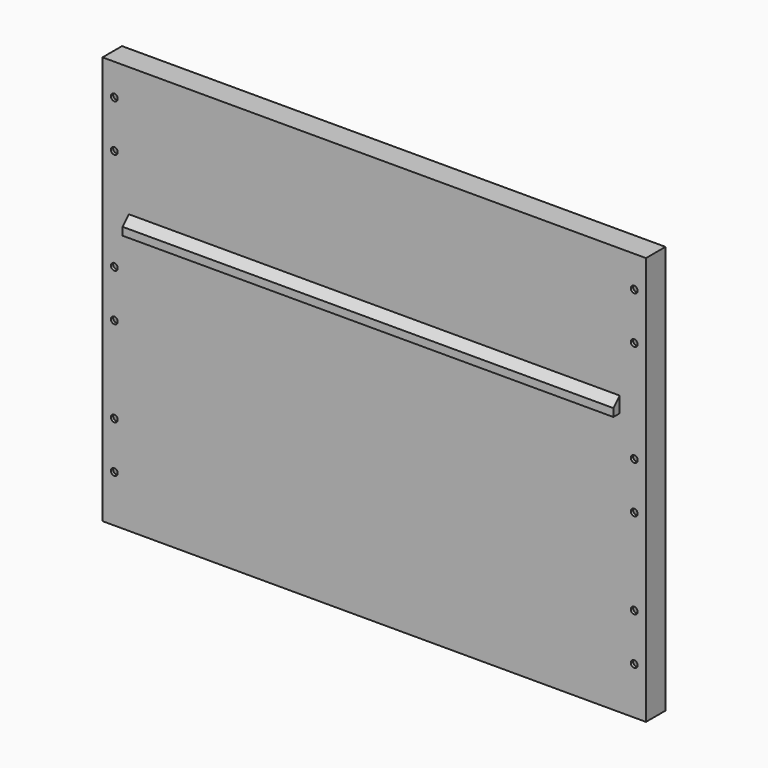
from build123d import *

# Parameters (mm, degrees)
F1_W           = 76.2
F1_H           = 76.2
F1_W_2         = 63.5
F1_H_2         = 63.5
F3_W           = 76.2
F3_H           = 76.2
F3_W_2         = 63.5
F3_H_2         = 63.5
F4_DEPTH       = 802.767
F4_DEPTH_BACK  = 802.767
F5_W           = 1757.934
F5_H           = 2.667
F6_DEPTH       = 660.4
F6_DEPTH_BACK  = 660.4
F7_W           = 19.05
F7_H           = 19.05
F8_DEPTH       = 793.75
F9_W           = 6.35
F9_H           = 25.4
F10_REACH      = 496.0827207226
F11_R          = 11.1125
F12_DEPTH      = 104.268
F13_R          = 9.525
F14_DEPTH      = 76.2
F15_R          = 6.35
F16_DEPTH      = 177.8
F16_DEPTH_BACK = 177.8


# Not quite as in the source:
# - an extrude ends at something that could not be found from the text; its depth is read off the source's solid


with BuildPart() as f2:
    # F2: sweep along a path in F0
    with BuildLine(Plane.XZ) as f2_path:
        Line((-878.967, 660.4), (878.967, 660.4))
        Line((878.967, 660.4), (878.967, -660.4))
        Line((878.967, -660.4), (-878.967, -660.4))
        Line((-878.967, -660.4), (-878.967, 660.4))
    # F1 (on Top) → F2 (sweep)
    with BuildSketch(Plane.XY):
        with Locations((-840.867, -38.1)):
            Rectangle(F1_W, F1_H)
        with Locations((-840.867, -38.1)):
            Rectangle(F1_W_2, F1_H_2, mode=Mode.SUBTRACT)
    sweep(path=f2_path.line, transition=Transition.RIGHT)

    # F3 (on Right) → F4 (join, two sides)
    with BuildSketch(Plane.YZ) as f4_sk:
        with Locations((-38.1, 215.9)):
            Rectangle(F3_W, F3_H)
        with Locations((-38.1, 215.9)):
            Rectangle(F3_W_2, F3_H_2, mode=Mode.SUBTRACT)
        with Locations((-38.1, -215.9)):
            Rectangle(F3_W, F3_H)
        with Locations((-38.1, -215.9)):
            Rectangle(F3_W_2, F3_H_2, mode=Mode.SUBTRACT)
    extrude(amount=-F4_DEPTH)
    extrude(f4_sk.sketch, amount=F4_DEPTH_BACK)

    # F5 (on Top) → F6 (join, two sides)
    with BuildSketch(Plane.XY) as f6_sk:
        with Locations((0, -77.5335)):
            Rectangle(F5_W, F5_H)
    extrude(amount=F6_DEPTH)
    extrude(f6_sk.sketch, amount=-F6_DEPTH_BACK)

    # F7 (on Right) → F8 (join, symmetric)
    with BuildSketch(Plane.YZ):
        Polygon((-78.867, 190.5), (-78.867, 215.9), (-102.5499750297, 215.9), (-104.267, 215.9), (-104.267, 190.5), align=None)
        with Locations((-91.567, 203.2)):
            Rectangle(F7_W, F7_H, mode=Mode.SUBTRACT)
        Polygon((-104.267, 215.9), (-102.5499750297, 215.9), (-78.867, 239.5829750297), (-78.867, 241.3), align=None)
    extrude(amount=F8_DEPTH, both=True)

    f10_end = Plane(origin=(0, -90.7084875148, 227.7414875149), x_dir=(0, 0.7071067812, 0.7071067812), z_dir=(0, 0.7071067812, -0.7071067812))
    # F9 (on face) → F10 (join, up to a plane its end follows)
    with BuildSketch(Plane(origin=(0, 0, 190.5000000001), x_dir=(1, 0, 0), z_dir=(0, 0, -1))):
        with Locations((790.575, 91.567)):
            Rectangle(F9_W, F9_H)
        with Locations((-790.575, 91.567)):
            Rectangle(F9_W, F9_H)
    f10_long = extrude(amount=-F10_REACH, mode=Mode.PRIVATE)
    add(split(f10_long, bisect_by=f10_end, keep=Keep.TOP, mode=Mode.PRIVATE))

    # F11 (on Front) → F12 (cut, through all)
    with BuildSketch(Plane.XZ):
        with Locations((-840.867, -76.2)):
            Circle(F11_R)
        with Locations((-840.867, -508)):
            Circle(F11_R)
        with Locations((-840.867, 76.2000000001)):
            Circle(F11_R)
        with Locations((-840.867, -355.6)):
            Circle(F11_R)
        with Locations((-840.867, 406.4)):
            Circle(F11_R)
        with Locations((-840.867, 558.8)):
            Circle(F11_R)
        with Locations((840.867, 558.8)):
            Circle(F11_R)
        with Locations((840.867, 406.4)):
            Circle(F11_R)
        with Locations((840.867, 76.2000000001)):
            Circle(F11_R)
        with Locations((840.867, -76.2)):
            Circle(F11_R)
        with Locations((840.867, -355.6)):
            Circle(F11_R)
        with Locations((840.867, -508)):
            Circle(F11_R)
    extrude(amount=F12_DEPTH, mode=Mode.SUBTRACT)

    # F13 (on face) → F14 (cut, through all)
    with BuildSketch(Plane.XY.offset(254)):
        with Locations((-726.567, -38.1)):
            Circle(F13_R)
        with Locations((726.567, -38.1)):
            Circle(F13_R)
    extrude(amount=-F14_DEPTH, mode=Mode.SUBTRACT)

    # F15 (on Top) → F16 (join, two sides)
    with BuildSketch(Plane.XY) as f16_sk:
        with Locations((-650.367, -12.7)):
            Circle(F15_R)
    extrude(amount=F16_DEPTH)
    extrude(f16_sk.sketch, amount=-F16_DEPTH_BACK)


solid = f2.part
